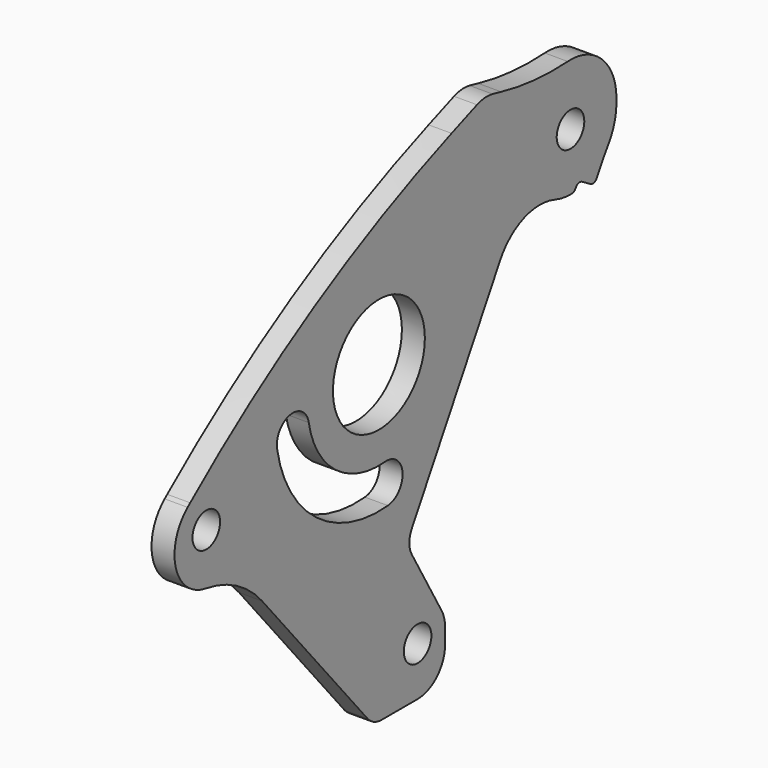
from build123d import *

# Parameters (mm, degrees)
F0_R     = 1.5
F0_R_2   = 5
F1_DEPTH = 2
F2_SCALE = 10


# Not quite as in the source:
# - ends of sketch curves that miss each other by under 0.0002 mm in the source are joined


with BuildPart() as f1:
    # F0 (on Right) → F1 (new body)
    with BuildSketch(Plane.YZ):
        with BuildLine():
            Line((20.303062, 10.815357), (21.213073, 10.271883))
            ThreePointArc((21.213073, 10.271883), (21.5939035848, 10.2168943828), (21.901025054, 10.4486959684))
            Line((21.901025054, 10.4486959684), (22.426599, 11.34717))
            ThreePointArc((22.426599, 11.34717), (22.7903712384, 11.9448053837), (23.1748242578, 12.529351507))
            ThreePointArc((23.1748242578, 12.529351507), (23.8232826043, 13.8736711803), (24.046052, 15.349499))
            Line((24.046052, 15.349499), (24.046052, 15.676385))
            ThreePointArc((24.046052, 15.676385), (22.4727964344, 19.3174593718), (18.7430829675, 20.6671975356))
            ThreePointArc((18.7430829675, 20.6671975356), (15.0971647826, 20.7122553198), (11.4965779735, 21.2871678873))
            ThreePointArc((11.4965779735, 21.2871678873), (11.0304932137, 21.3939885254), (10.5631540495, 21.4951802352))
            ThreePointArc((10.5631540495, 21.4951802352), (9.7072570471, 21.5498382875), (8.8708699259, 21.360092193))
            Line((8.8708699259, 21.360092193), (6.103052, 20.297626))
            ThreePointArc((6.103052, 20.297626), (-8.8139895114, 13.1024999173), (-22.3389141406, 3.5440281676))
            Line((-22.3389141406, 3.5440281676), (-22.617202, 3.310517))
            ThreePointArc((-22.617202, 3.310517), (-23.8982246357, -0.8310495022), (-20.6544870079, -3.7071160511))
            ThreePointArc((-20.6544870079, -3.7071160511), (-17.2704039619, -4.8764379221), (-14.5151312861, -7.1628772401))
            Line((-14.5151312861, -7.1628772401), (-3.03453, -20.844925))
            ThreePointArc((-3.03453, -20.844925), (-2.3476776328, -21.3719655231), (-1.502441, -21.55935))
            Line((-1.502441, -21.55935), (2.405537, -21.55935))
            ThreePointArc((2.405537, -21.55935), (4.5268573436, -20.6806703436), (5.405537, -18.55935))
            Line((5.405537, -18.55935), (5.405537, -17.30935))
            ThreePointArc((5.405537, -17.30935), (5.3033144652, -16.5328928137), (5.0036131585, -15.8093499085))
            Line((5.0036131585, -15.8093499085), (1.781026, -10.227666))
            ThreePointArc((1.781026, -10.227666), (1.513077, -9.227666), (1.7810261443, -8.2276660833))
            Line((1.7810261443, -8.2276660833), (11.391549, 8.418247))
            ThreePointArc((11.391549, 8.418247), (13.9876851036, 10.6079458785), (17.3838640825, 10.633873234))
            ThreePointArc((17.3838640825, 10.633873234), (18.2706804185, 10.4099849641), (19.1834430004, 10.3513869851))
            ThreePointArc((19.1834430004, 10.3513869851), (19.4332447525, 10.4262916315), (19.6113513075, 10.6167898368))
            ThreePointArc((19.6113513075, 10.6167898368), (19.9150373869, 10.862970839), (20.303062, 10.815357))
        make_face()
        with Locations((2.405537, -17.30935)):
            Circle(F0_R, mode=Mode.SUBTRACT)
        with Locations((-20.58619, 0.760036)):
            Circle(F0_R, mode=Mode.SUBTRACT)
        with BuildLine():
            ThreePointArc((-0.8233559685, -5.41610236), (-8.6524240902, -3.1341370676), (-12.8829452145, 3.8375459622))
            ThreePointArc((-12.8829452145, 3.8375459622), (-11.4634165059, 5.8648445334), (-9.436118366, 4.4453149355))
            ThreePointArc((-9.436118366, 4.4453149355), (-6.5217592217, -0.3574002745), (-1.1284010077, -1.9294209114))
            ThreePointArc((-1.1284010077, -1.9294209114), (0.7674627243, -3.5202384804), (-0.8233559685, -5.41610236))
        make_face(mode=Mode.SUBTRACT)
        with Locations((-1.803858, 5.791088)):
            Circle(F0_R_2, mode=Mode.SUBTRACT)
        with Locations((19.046052, 15.349499)):
            Circle(F0_R, mode=Mode.SUBTRACT)
    extrude(amount=F1_DEPTH)


with BuildPart() as f1_1:
    # F2: moved
    add(f1.part.scale(F2_SCALE).moved(Location((0, 185.27571, -6.840324))))


solid = f1_1.part
